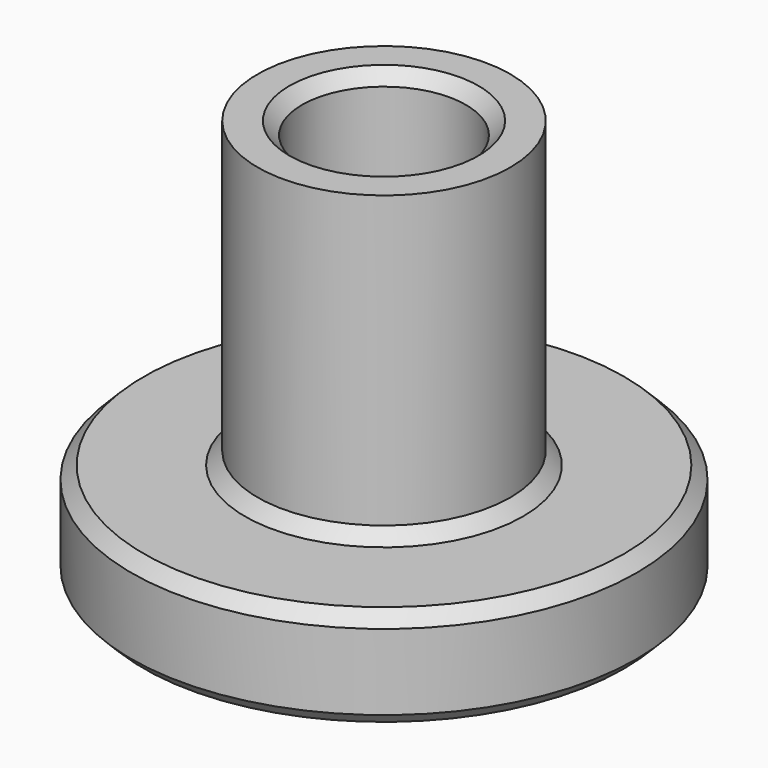
from build123d import *

# Parameters (mm, degrees)
F0_R     = 15.875
F1_DEPTH = 25.4
F2_D     = 10.3
F3_SIZE  = 0.79375
F4_SIZE  = 0.79375
F5_R     = 15.875
F5_R_2   = 7.9375
F6_DEPTH = 19.05
F7_SIZE  = 0.79375


with BuildPart() as f1:
    # F0 (on Top) → F1 (new body)
    with BuildSketch(Plane.XY):
        Circle(F0_R)
    extrude(amount=F1_DEPTH)

    # F2 (through all)
    with Locations(Plane(origin=(0, 0, 0), x_dir=(1, 0, 0), z_dir=(0, 0, -1))):
        with Locations((0, 0)):
            Hole(F2_D / 2)

    # F3
    f3_edges = [f1.edges().sort_by_distance(p)[0] for p in [
        (-15.875, 0, 0),
    ]]
    chamfer(f3_edges, length=F3_SIZE)

    # F4
    f4_edges = [f1.edges().sort_by_distance(p)[0] for p in [
        (-15.875, 0, 25.4),
        (-5.15, 0, 25.4),
        (-5.15, 0, 0),
    ]]
    chamfer(f4_edges, length=F4_SIZE)

    # F5 (on face) → F6 (cut)
    with BuildSketch(Plane.XY.offset(25.4)):
        Circle(F5_R)
        Circle(F5_R_2, mode=Mode.SUBTRACT)
    extrude(amount=-F6_DEPTH, mode=Mode.SUBTRACT)

    # F7
    f7_edges = [f1.edges().sort_by_distance(p)[0] for p in [
        (-15.875, 0, 6.35),
        (-7.9375, 0, 6.35),
    ]]
    chamfer(f7_edges, length=F7_SIZE)


solid = f1.part
